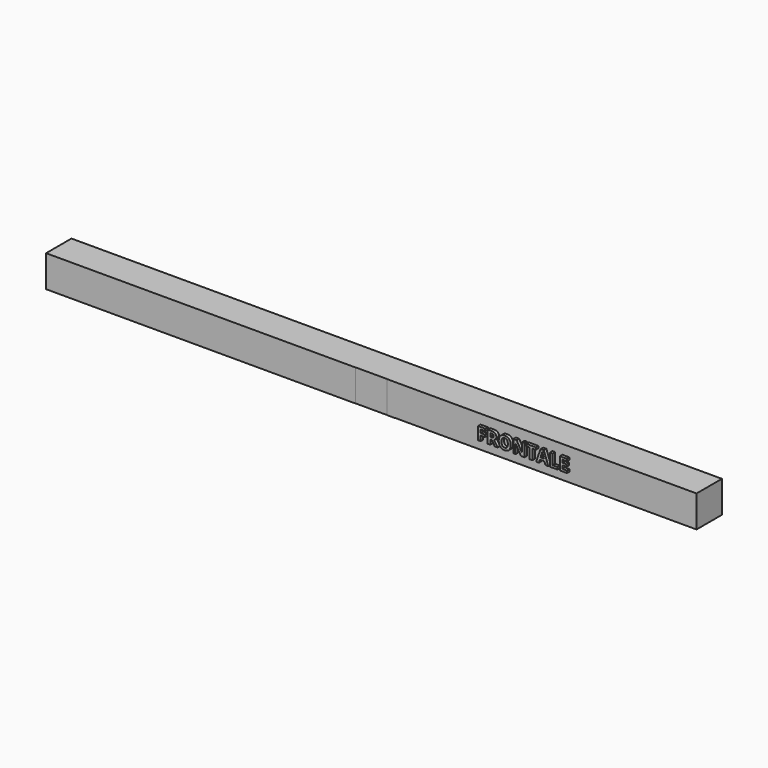
from build123d import *

# Parameters (mm, degrees)
F0_W         = 410
F0_H         = 20
F1_DEPTH     = 20
F3_TEXT_SIZE = 11.072636375
F4_DEPTH     = 2
F2_W         = 20
F2_H         = 20
F6_DEPTH     = 0.1
F5_W         = 20
F5_H         = 20
F7_DEPTH     = 0.1


# Not quite as in the source:
# - Text() gives the source's letters only with a copy of the font that has no kerning and outlines rounded to 1/6400 em; it was checked with that copy


with BuildPart() as f1:
    # F0 (on Front) → F1 (new body)
    with BuildSketch(Plane.XZ):
        with Locations((59.9894565077, 15.8952437341)):
            Rectangle(F0_W, F0_H)
    extrude(amount=F1_DEPTH)

    # F3 (on face) → F4 (join)
    with BuildSketch(Plane.XZ.offset(20)):
        with Locations((127.8745681047, 11.9744390249)):
            Text('FRONTALE', F3_TEXT_SIZE, font='Open Sans', font_style=FontStyle.BOLD, text_align=(TextAlign.LEFT, TextAlign.BOTTOM))
    extrude(amount=F4_DEPTH)

    # F2 (on face) → F6 (cut)
    with BuildSketch(Plane.XZ.offset(20)):
        with Locations((59.9894565077, 15.8952437341)):
            Rectangle(F2_W, F2_H)
    extrude(amount=-F6_DEPTH, mode=Mode.SUBTRACT)

    # F5 (on face) → F7 (cut)
    with BuildSketch(Plane(origin=(0, 0, 5.8952437341), x_dir=(1, 0, 0), z_dir=(0, 0, -1))):
        with Locations((84.9894565077, 10)):
            Rectangle(F5_W, F5_H)
    extrude(amount=-F7_DEPTH, mode=Mode.SUBTRACT)


solid = f1.part
